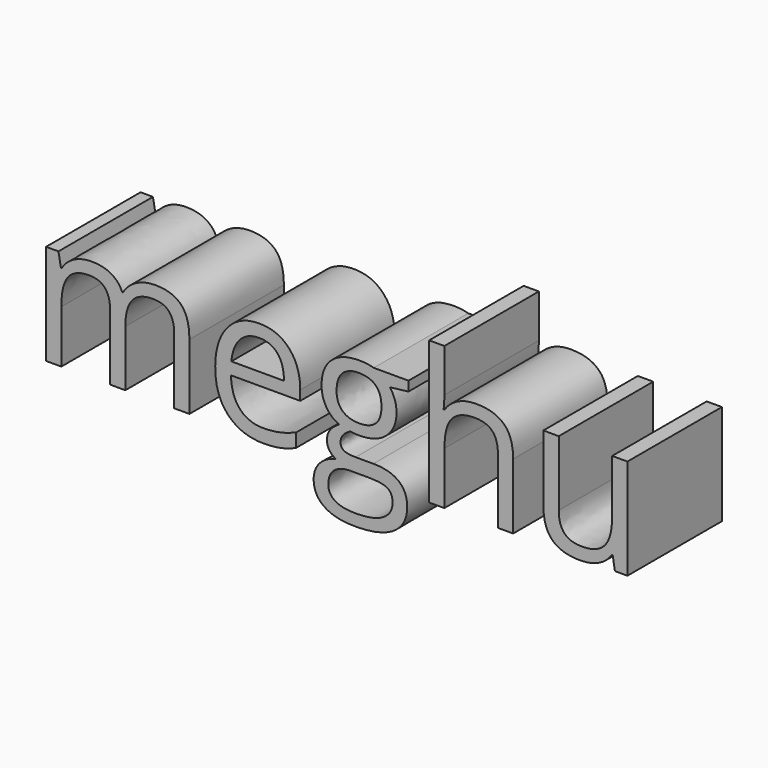
from build123d import *

# Parameters (mm, degrees)
F0_TEXT_SIZE = 39.7654560705
F1_DEPTH     = 25


# Not quite as in the source:
# - Text() gives the source's letters only with a copy of the font that has no kerning and outlines rounded to 1/6400 em; it was checked with that copy


with BuildPart() as f1:
    # F0 (on Front) → F1 (new body)
    with BuildSketch(Plane.XZ):
        with Locations((-47.3845824599, 34.7958281636)):
            Text('meghu', F0_TEXT_SIZE, font='Open Sans', text_align=(TextAlign.LEFT, TextAlign.BOTTOM))
    extrude(amount=F1_DEPTH)


solid = f1.part
